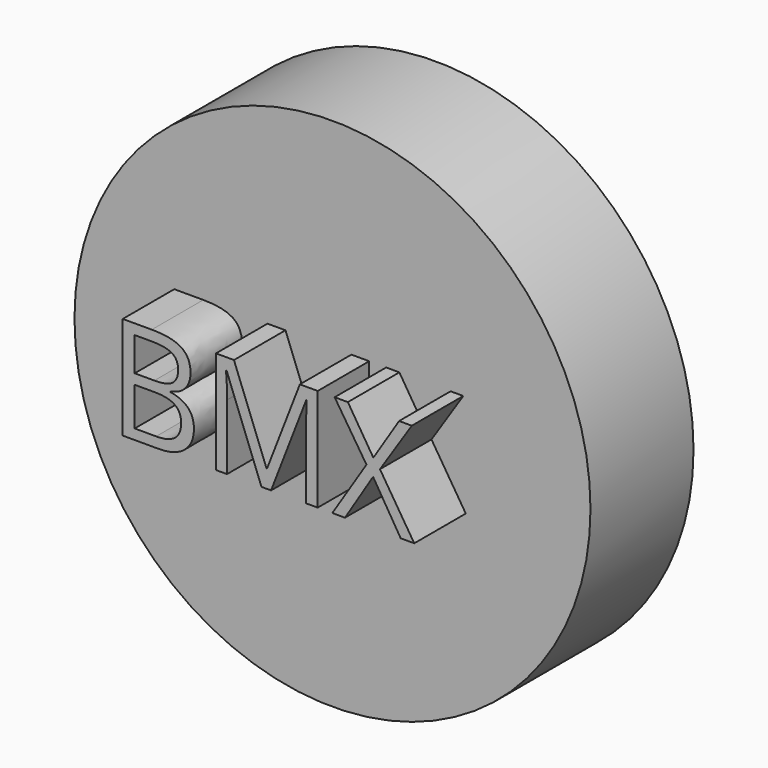
from build123d import *

# Parameters (mm, degrees)
F1_TEXT_SIZE = 28.3779848057
F2_DEPTH     = 38.1
F0_R         = 50.8846685463
F3_DEPTH     = 25.4


# Not quite as in the source:
# - Text() gives the source's letters only with a copy of the font that has no kerning and outlines rounded to 1/6400 em; it was checked with that copy


with BuildPart() as f2:
    # F1 (on face) → F2 (new body)
    with BuildSketch(Plane.XZ):
        with Locations((-33.9899286628, -8.7839141488)):
            Text('BMX', F1_TEXT_SIZE, font='Open Sans', text_align=(TextAlign.LEFT, TextAlign.BOTTOM))
    extrude(amount=F2_DEPTH)


with BuildPart() as f3:
    # F0 (on Front) → F3 (new body)
    with BuildSketch(Plane.XZ):
        Circle(F0_R)
    extrude(amount=F3_DEPTH)


solid = Compound([f2.part, f3.part])
